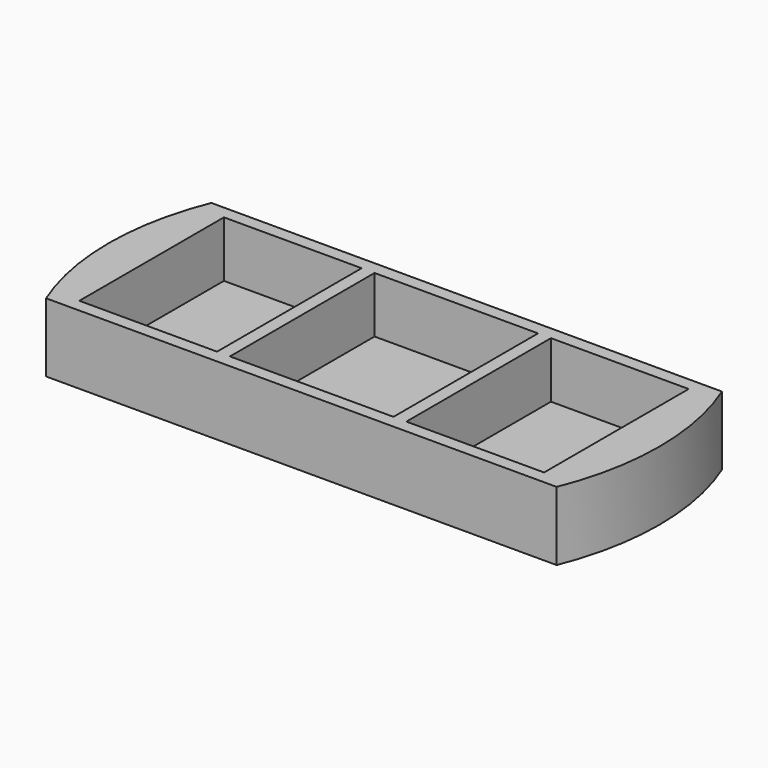
from build123d import *

# Parameters (mm, degrees)
F0_W     = 203.2
F0_H     = 25.4
F1_DEPTH = 76.2
F3_DEPTH = 25.4
F4_W     = 30.1625
F4_H     = 66.675
F5_DEPTH = 20.6375


with BuildPart() as f1:
    # F0 (on Front) → F1 (new body)
    with BuildSketch(Plane.XZ):
        with Locations((-101.6, 12.7)):
            Rectangle(F0_W, F0_H)
    extrude(amount=F1_DEPTH)

    # F2 (on face) → F3 (cut)
    with BuildSketch(Plane.XY.offset(25.4)):
        with BuildLine():
            Line((0, -76.2), (0, -38.1))
            ThreePointArc((0, -38.1), (-1.8707935661, -57.5073538656), (-7.4142792139, -76.2))
            Line((-7.4142792139, -76.2), (0, -76.2))
        make_face()
        with BuildLine():
            ThreePointArc((-7.4142792139, 0), (-1.8707935661, -18.6926461344), (0, -38.1))
            Line((0, -38.1), (0, 0))
            Line((0, 0), (-7.4142792139, 0))
        make_face()
        with BuildLine():
            ThreePointArc((-195.7857207861, -76.2), (-101.6, -139.7), (-7.4142792139, -76.2))
            Line((-7.4142792139, -76.2), (-195.7857207861, -76.2))
        make_face()
        with BuildLine():
            ThreePointArc((-203.2, -38.1), (-201.3292064339, -18.6926461344), (-195.7857207861, 0))
            Line((-195.7857207861, 0), (-203.2, 0))
            Line((-203.2, 0), (-203.2, -38.1))
        make_face()
        with BuildLine():
            Line((-203.2, -76.2), (-195.7857207861, -76.2))
            ThreePointArc((-195.7857207861, -76.2), (-201.3292064339, -57.5073538656), (-203.2, -38.1))
            Line((-203.2, -38.1), (-203.2, -76.2))
        make_face()
    extrude(amount=-F3_DEPTH, mode=Mode.SUBTRACT)

    # F4 (on face) → F5 (cut)
    with BuildSketch(Plane.XY.offset(25.4)):
        Polygon((-187.325, -4.7625), (-187.325, -38.1), (-187.325, -71.4375), (-136.525, -71.4375), (-136.525, -4.7625), align=None)
        Polygon((-15.875, -71.4375), (-15.875, -38.1), (-15.875, -4.7625), (-66.675, -4.7625), (-66.675, -71.4375), align=None)
        with Locations((-86.51875, -38.1)):
            Rectangle(F4_W, F4_H)
        with Locations((-116.68125, -38.1)):
            Rectangle(F4_W, F4_H)
    extrude(amount=-F5_DEPTH, mode=Mode.SUBTRACT)


solid = f1.part
